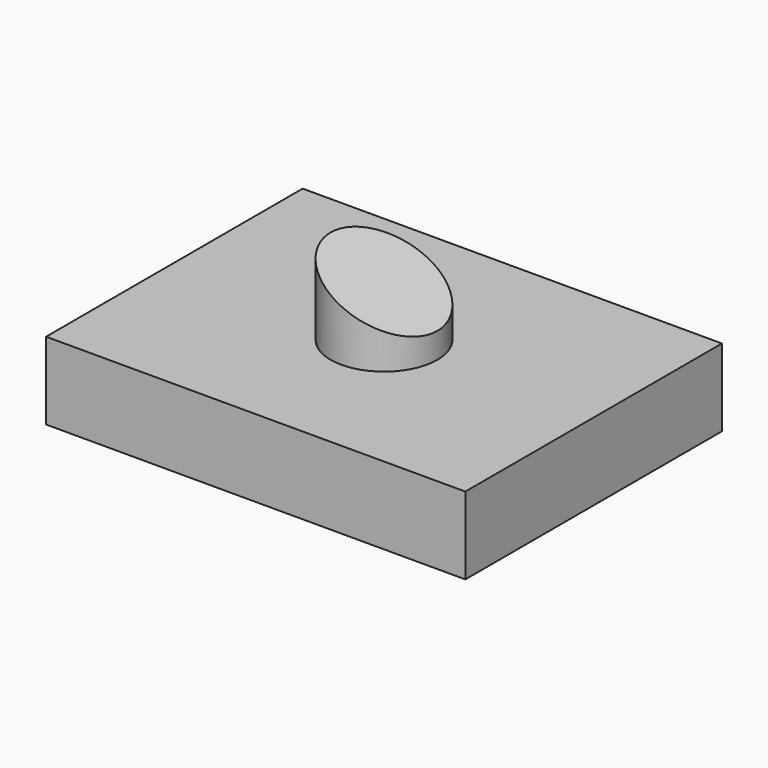
from build123d import *

# Parameters (mm, degrees)
F0_W     = 135.5276703835
F0_H     = 103.6717817187
F1_DEPTH = 25
F2_R     = 17.2700021185
F3_DEPTH = 25
F5_DEPTH = 103.6727817187


# Not quite as in the source:
# - a feature names something its author has since deleted; it is built from what else it names


with BuildPart() as f1:
    # F0 (on Top) → F1 (new body)
    with BuildSketch(Plane.XY):
        Rectangle(F0_W, F0_H)
    extrude(amount=F1_DEPTH)

    # F2 (on face) → F3 (join)
    with BuildSketch(Plane.XY.offset(25)):
        Circle(F2_R)
    extrude(amount=F3_DEPTH)

    # F4 (on face) → F5 (cut, through all)
    with BuildSketch(Plane.XZ.offset(51.8358908594)):
        Polygon((23.7591248006, 58.1170134246), (-17.2700021185, 50), (17.2700021185, 33.2325548289), (23.7591248006, 30.0824102014), align=None)
    extrude(amount=-F5_DEPTH, mode=Mode.SUBTRACT)


solid = f1.part
